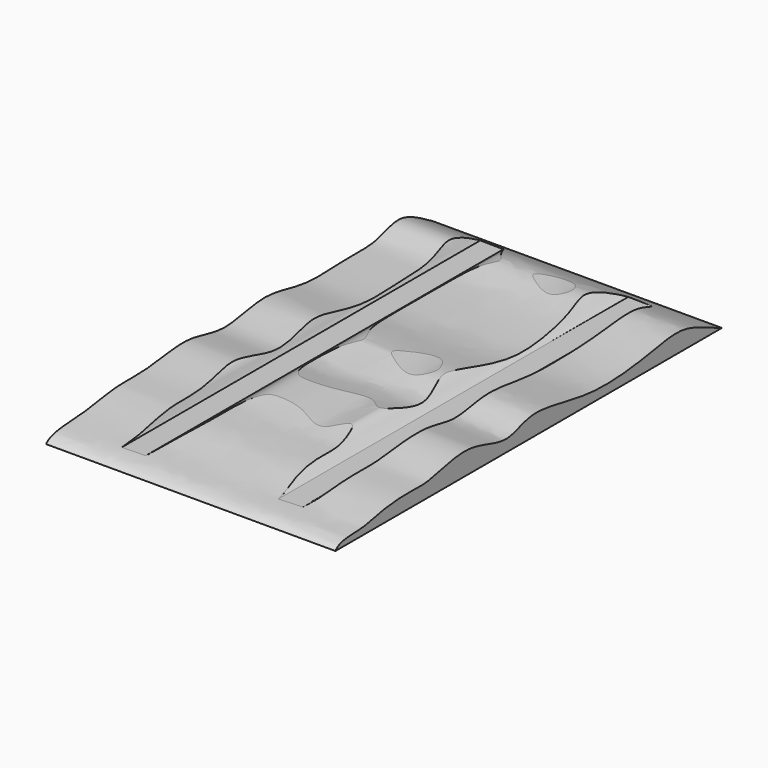
from build123d import *

# Parameters (mm, degrees)
F8_DEPTH = 206.2010001


with BuildPart() as f6:
    # F4 (on plane+point) → F6 section 0
    with BuildSketch(Plane.YZ.offset(61.75)):
        with BuildLine():
            Line((-103.1, 0), (103.1, 0))
            add(Edge.make_bspline(
                [(-103.1, 0), (-100.9122427395, 3.0077628671), (-88.9320477254, 2.1674578087), (-79.9375830942, 5.1227732359), (-64.1648905521, 6.5195980018), (-53.3351288094, 5.1288378697), (-32.0364127365, 12.6659806153), (-11.8976279776, 1.9219681319), (1.7800190529, 11.6036150432), (32.5487128992, 1.5761209838), (64.9509129805, 5.8214608578), (83.6967649592, 9.8765664291), (96.9200083349, 2.2529806795), (103.1, 0)],
                knots=[0, 0, 0, 0, 0.0775712537, 0.1470290462, 0.2285878895, 0.2995643402, 0.3975281521, 0.4936065892, 0.5729404733, 0.6906593695, 0.8127041165, 0.903754243, 1, 1, 1, 1], degree=3))
        make_face()
    # F5 (on plane+point) → F6 section 1
    with BuildSketch(Plane.YZ.offset(-61.75)):
        with BuildLine():
            Line((-103.1, 0), (103.1, 0))
            add(Edge.make_bspline(
                [(103.1, 0), (97.6939418577, 3.0688433364), (86.0835229647, 10.7763185605), (73.3931731646, 3.7067739886), (56.2353160284, 4.9215645971), (34.3821378247, 2.7288399062), (13.4519982501, 10.2069669537), (-8.3349312407, 2.5879784187), (-27.0423994972, 10.4843331765), (-48.2959652127, 5.6165498905), (-66.7498639179, 6.9726497282), (-82.8586426999, 2.9062747734), (-100.4594381736, 3.3068484577), (-103.1, 0)],
                knots=[0, 0, 0, 0, 0.0906610015, 0.1654943193, 0.2511327642, 0.3489868085, 0.4462251661, 0.5432237858, 0.6349895725, 0.7312170544, 0.8198077577, 0.9087646464, 1, 1, 1, 1], degree=3))
        make_face()
    loft()

    # F7 (on plane+point) → F8 (cut, through all)
    with BuildSketch(Plane.XZ.offset(103.1)):
        with BuildLine():
            Line((-61.75, 26.2276791036), (-61.75, 12.6142017543))
            add(Edge.make_bspline(
                [(-37, 3), (-37.9685674323, 4.1927412246), (-38.6449691785, 11.1950543754), (-53.9987916753, 8.0543119967), (-58.7080877818, 12.3875886996), (-61.75, 12.6142017543)],
                knots=[0, 0, 0, 0, 0.2736754451, 0.6693012904, 1, 1, 1, 1], degree=3))
            Line((-37, 3), (-27, 3))
            add(Edge.make_bspline(
                [(-27, 3), (-25.683950102, 3.7041694158), (-21.4001922621, 7.7696799402), (-12.6726198769, 8.0063626166), (0.2479387085, 7.8751023452), (12.079651288, 6.3463341801), (20.7085255522, 9.8282843188), (24.7019248278, 3.868789004), (27, 3)],
                knots=[0, 0, 0, 0, 0.1403791106, 0.3013484227, 0.4992568681, 0.6893819706, 0.843449848, 1, 1, 1, 1], degree=3))
            Line((27, 3), (37, 3))
            add(Edge.make_bspline(
                [(37, 3), (37.6001875911, 3.3094298489), (39.2495556594, 4.1597701757), (40.8080605464, 12.8272863702), (52.84418989, 11.7031358222), (61.5861332452, 14.0803504545), (61.75, 13.9561323449)],
                knots=[0, 0, 0, 0, 0.1406039588, 0.3863919937, 0.713664837, 0.982511832, 0.982511832, 0.982511832, 0.982511832], degree=3))
            Line((61.75, 13.9561323449), (61.75, 26.2276791036))
            Line((61.75, 26.2276791036), (-61.75, 26.2276791036))
        make_face()
    extrude(amount=-F8_DEPTH, mode=Mode.SUBTRACT)


solid = f6.part
